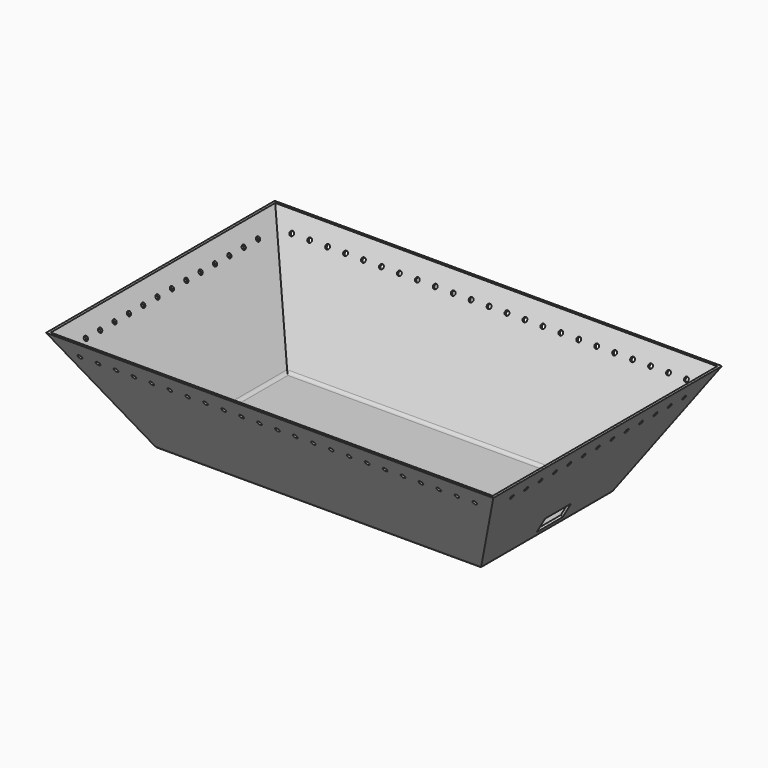
from build123d import *

# Parameters (mm, degrees)
F0_W                   = 914.4
F0_H                   = 457.2
F1_DEPTH               = 304.8
DRAFT_F1_DRAFTED_ANGLE = -30
F2_T                   = -6.35
F7_D                   = 12.7
F7_ON_F4_D             = 12.7
F7_ON_F5_D             = 12.7
F7_ON_F6_D             = 12.7
F8_R                   = 12.7
F9_R                   = 19.05
F10_W                  = 92.075
F10_H                  = 47.66056
F11_DEPTH              = 2050


# Not quite as in the source:
# - an extrude ends at something that could not be found from the text; its depth is read off the source's solid
# - an extrude with a draft is written as a straight extrude whose walls are then drafted


with BuildPart() as f1:
    # F0 (on Top) → F1 (new body)
    with BuildSketch(Plane.XY):
        with Locations((0, -228.6)):
            Rectangle(F0_W, F0_H)
    extrude(amount=F1_DEPTH)

    # draft_F1_drafted
    draft_f1_drafted_walls = [f1.faces().sort_by_distance(p)[0] for p in [
        (-457.2, -228.6, 203.2),
        (0, -457.2, 203.2),
        (457.2, -228.6, 203.2),
        (0, 0, 203.2),
    ]]
    draft(draft_f1_drafted_walls, neutral_plane=Plane.XY, angle=DRAFT_F1_DRAFTED_ANGLE)

    # F2
    f2_openings = [f1.faces().sort_by_distance(p)[0] for p in [
        (0, -228.6, 304.8),
    ]]
    offset(amount=F2_T, openings=f2_openings)

    # F7 (through all)
    with Locations(Plane(origin=(0, -5.499261314, 3.175), x_dir=(1, 0, 0), z_dir=(0, -0.8660254038, 0.5))):
        with Locations((0, 297.4865498886), (50.8, 297.4865498886), (101.6, 297.4865498886), (152.4, 297.4865498886), (203.2, 297.4865498886), (254, 297.4865498886), (-50.8, 297.4865498886), (-101.6, 297.4865498886), (-152.4, 297.4865498886), (-203.2, 297.4865498886), (-254, 297.4865498886), (508, 297.4865498886), (304.8, 297.4865498886), (355.6, 297.4865498886), (457.2, 297.4865498886), (406.4, 297.4865498886), (558.8, 297.4865498886), (-457.2, 297.4865498886), (-558.8, 297.4865498886), (-508, 297.4865498886), (-406.4, 297.4865498886), (-304.8, 297.4865498886), (-355.6, 297.4865498886)):
            Hole(F7_D / 2)

    # F7 on F4 (through all)
    with Locations(Plane(origin=(0, -337.400738686, -194.7984073051), x_dir=(-1, 0, 0), z_dir=(0, 0.8660254038, 0.5))):
        with Locations((-254, 526.0865498886), (-203.2, 526.0865498886), (-152.4, 526.0865498886), (-101.6, 526.0865498886), (-50.8, 526.0865498886), (0, 526.0865498886), (50.8, 526.0865498886), (101.6, 526.0865498886), (152.4, 526.0865498886), (203.2, 526.0865498886), (254, 526.0865498886), (-304.8, 526.0865498886), (-355.6, 526.0865498886), (-406.4, 526.0865498886), (-457.2, 526.0865498886), (-508, 526.0865498886), (-558.8, 526.0865498886), (457.2, 526.0865498886), (558.8, 526.0865498886), (558.8, 526.0865498886), (508, 526.0865498886), (406.4, 526.0865498886), (355.6, 526.0865498886), (304.8, 526.0865498886)):
            Hole(F7_ON_F4_D / 2)

    # F7 on F5 (through all)
    with Locations(Plane(origin=(-337.400738686, 0, -194.7984073051), x_dir=(0, 1, 0), z_dir=(0.8660254038, 0, 0.5))):
        with Locations((-533.4, 526.0865498886), (-482.6, 526.0865498886), (-431.8, 526.0865498886), (-381, 526.0865498886), (-330.2, 526.0865498886), (-279.4, 526.0865498886), (-228.6, 526.0865498886), (-177.8, 526.0865498886), (-127, 526.0865498886), (-76.2, 526.0865498886), (-25.4, 526.0865498886), (25.4, 526.0865498886), (76.2, 526.0865498886)):
            Hole(F7_ON_F5_D / 2)

    # F7 on F6 (through all)
    with Locations(Plane(origin=(337.400738686, 0, -194.7984073051), x_dir=(0, -1, 0), z_dir=(-0.8660254038, 0, 0.5))):
        with Locations((-76.2, 526.0865498886), (-25.4, 526.0865498886), (25.4, 526.0865498886), (76.2, 526.0865498886), (127, 526.0865498886), (177.8, 526.0865498886), (228.6, 526.0865498886), (279.4, 526.0865498886), (330.2, 526.0865498886), (381, 526.0865498886), (431.8, 526.0865498886), (482.6, 526.0865498886), (533.4, 526.0865498886)):
            Hole(F7_ON_F6_D / 2)

    # F8
    f8_edges = [f1.edges().sort_by_distance(p)[0] for p in [
        (453.533826, -228.6, 6.35),
        (0, -3.666174, 6.35),
        (0, -453.533826, 6.35),
        (-453.533826, -228.6, 6.35),
    ]]
    fillet(f8_edges, radius=F8_R)

    # F9
    f9_edges = [f1.edges().sort_by_distance(p)[0] for p in [
        (-457.2, -228.6, 0),
        (0, 0, 0),
        (0, -457.2, 0),
        (457.2, -228.6, 0),
    ]]
    fillet(f9_edges, radius=F9_R)

    # F10 (on face) → F11 (cut, through all)
    with BuildSketch(Plane(origin=(337.400738686, 0, -194.7984073051), x_dir=(0, -1, 0), z_dir=(-0.8660254038, 0, 0.5))):
        with Locations((228.6, 276.2558026281)):
            Rectangle(F10_W, F10_H)
    extrude(amount=-F11_DEPTH, mode=Mode.SUBTRACT)


solid = f1.part
